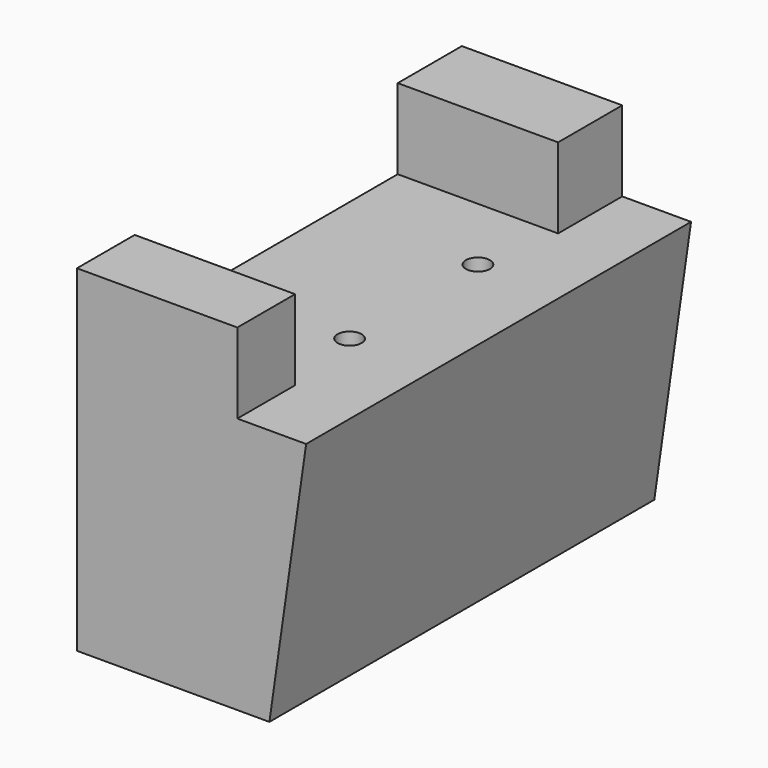
from build123d import *

# Parameters (mm, degrees)
F1_DEPTH = 30
F2_R     = 0.75
F3_DEPTH = 10
F4_W     = 10
F4_H     = 5
F4_H_2   = 4.5
F5_DEPTH = 5


# Not quite as in the source:
# - a feature names something its author has since deleted; it is built from what else it names


with BuildPart() as f1:
    # F0 (on Front) → F1 (new body)
    with BuildSketch(Plane.XZ):
        Polygon((0, 16), (0, 0), (12, 0), (14.29, 16), align=None)
    extrude(amount=F1_DEPTH)

    # F2 (on face) → F3 (cut)
    with BuildSketch(Plane.XY.offset(16)):
        with Locations((9, -10)):
            Circle(F2_R)
        with Locations((9, -20)):
            Circle(F2_R)
    extrude(amount=-F3_DEPTH, mode=Mode.SUBTRACT)

    # F4 (on face) → F5 (join)
    with BuildSketch(Plane.XY.offset(16)):
        with Locations((5, -2.5)):
            Rectangle(F4_W, F4_H)
        with Locations((5, -27.75)):
            Rectangle(F4_W, F4_H_2)
    extrude(amount=F5_DEPTH)


solid = f1.part
